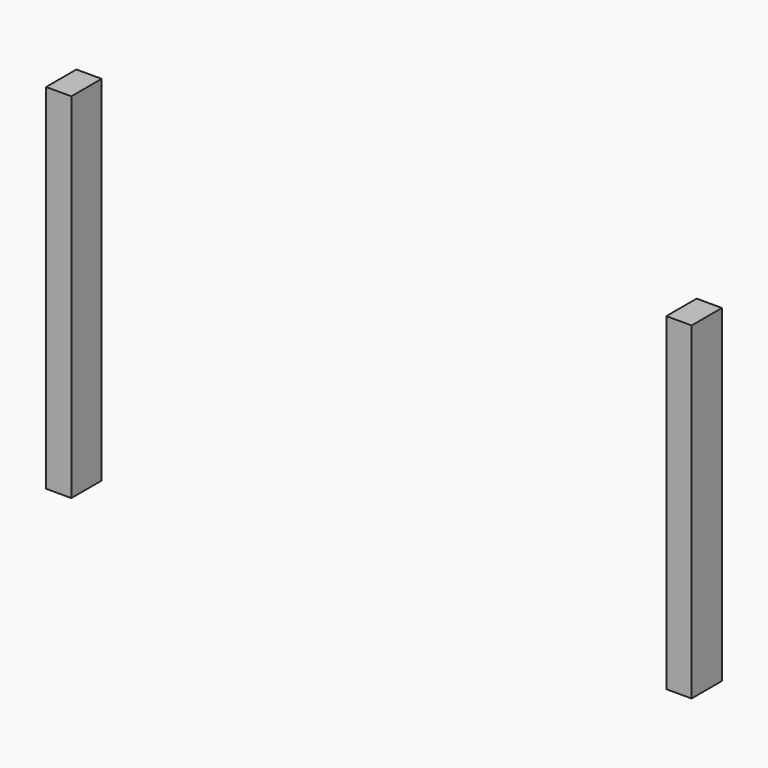
from build123d import *

# Parameters (mm, degrees)
F0_W     = 50.8
F0_H     = 76.2
F5_DEPTH = 711.2
F6_DEPTH = 660.4


# Not quite as in the source:
# - a feature of the source that left no trace in its solid (it failed there, or was rolled back) is left out


with BuildPart() as f5:
    # F0 (on Top) → F5 (new body)
    with BuildSketch(Plane.XY):
        with Locations((-623.57, 152.4)):
            Rectangle(F0_W, F0_H)
    extrude(amount=-F5_DEPTH)


with BuildPart() as f6:
    # F0 (on Top) → F6 (new body)
    with BuildSketch(Plane.XY):
        with Locations((623.57, 152.4)):
            Rectangle(F0_W, F0_H)
    extrude(amount=-F6_DEPTH)


solid = Compound([f5.part, f6.part])
